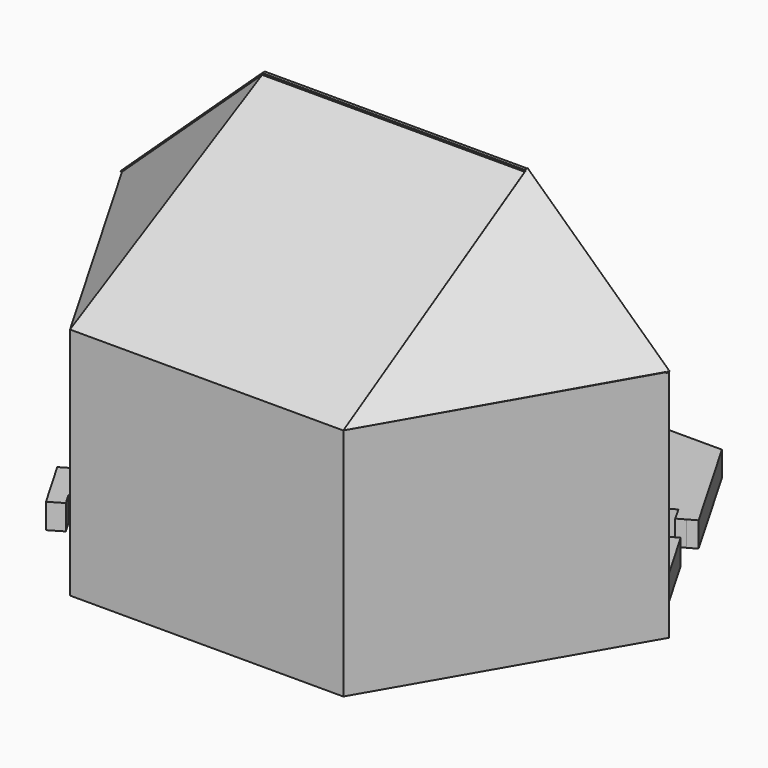
from build123d import *

# Parameters (mm, degrees)
F0_W      = 50
F0_H      = 12.5
F1_DEPTH  = 8
F2_DEPTH  = 75
F4_DEPTH  = 8
F7_DEPTH  = 3
F8_DEPTH  = 1
F11_DEPTH = 3
F14_DEPTH = 3
F15_DEPTH = 8
F16_DEPTH = 8


# Not quite as in the source:
# - a feature names something its author has since deleted; it is built from what else it names


with BuildPart() as f1:
    # F0 (on Top) → F1 (new body)
    with BuildSketch(Plane.XY):
        Polygon((57.9695070384, 39.3207329262), (60.5095952989, 40.7487522591), (42.0179491924, 72.7772228311), (-42.0179491924, 72.7772228311), (-84.0358983849, 0), (-42.0179491924, -72.7772228311), (42.0179491924, -72.7772228311), (84.0358983849, 0), (65.5097997054, 32.0881441788), (62.870004896, 30.6039762231), (65.3204122546, 26.2455930623), (60.0654171506, 23.2910848888), (57.615009792, 27.6494680496), (55.164720758, 32.0079177338), (52.7144317239, 36.366367418), (50.2642610162, 40.7248836223), (55.5194165334, 43.6791064608), align=None)
        with Locations((0, 54.5829171234)):
            Rectangle(F0_W, F0_H, mode=Mode.SUBTRACT)
    extrude(amount=F1_DEPTH)

    # F0 (on Top) → F2 (join)
    with BuildSketch(Plane.XY):
        Polygon((-84.0358983849, 0), (-87.5, 0), (-68.1246734519, -33.5590499945), (-63.1251610364, -42.2184595112), (-43.75, -75.7772228311), (43.75, -75.7772228311), (87.5, 0), (84.0358983849, 0), (42.0179491924, -72.7772228311), (-42.0179491924, -72.7772228311), align=None)
    extrude(amount=F2_DEPTH)

    # F0 (on Top) → F4 (join)
    with BuildSketch(Plane.XY):
        Polygon((43.75, 75.7772228311), (-43.75, 75.7772228311), (-65.625, 37.8886114156), (-68.125, 33.5584843966), (-87.5, 0), (-84.0358983849, 0), (-42.0179491924, 72.7772228311), (42.0179491924, 72.7772228311), (60.5095952989, 40.7487522591), (63.1248363216, 42.2190219338), align=None)
    extrude(amount=F4_DEPTH)

    # F6 (on face) → F7 (join)
    with BuildSketch(Plane(origin=(0, -50.1312366318, 89.3836679776), x_dir=(1, 0, 0), z_dir=(0, 0.4891706574, -0.872188092))):
        Polygon((43.75, 29.4041920927), (0, 29.4041920927), (-43.75, 29.4041920927), (-42.01795, -57.4775522498), (42.01795, -57.4775522498), align=None)
    extrude(amount=F7_DEPTH)

    # F3 (on Front) → F8 (join)
    with BuildSketch(Plane.XZ):
        Polygon((-42.01795, 114.5), (0, 114.5), (42.01795, 114.5), (84.0359, 75), (87.5, 75), (42.01795, 117.5), (0, 117.5), (-42.01795, 117.5), (-87.5, 75), (-84.0359, 75), align=None)
    extrude(amount=F8_DEPTH)

    # F10 (on face) → F11 (join)
    with BuildSketch(Plane(origin=(-67.6846727043, -39.0777640058, 72.4338274863), x_dir=(0.7723629594, -0.3015876344, 0.5590173143), z_dir=(-0.6351814378, -0.3667221741, 0.6797495039))):
        Polygon((33.2314262259, 55.789645187), (-25.6554603702, 35.6104118215), (30.9888924807, -31.0804218073), align=None)
    extrude(amount=-F11_DEPTH)

    # F13 (on face) → F14 (join)
    with BuildSketch(Plane(origin=(67.6756688636, -39.5950852503, 72.4241918832), x_dir=(0.7733047167, 0.3041472681, -0.556322078), z_dir=(-0.6340345536, 0.3709553614, -0.6785221475))):
        Polygon((-30.939509805, 30.5117392321), (-32.8751652468, -56.3649154418), (25.9400068576, -35.9776056011), align=None)
    extrude(amount=F14_DEPTH)

    # F0 (on Top) → F15 (join)
    with BuildSketch(Plane.XY):
        with Locations((0, 54.5829171234)):
            Rectangle(F0_W, F0_H)
    extrude(amount=F15_DEPTH)

    # F0 (on Top) → F16 (join)
    with BuildSketch(Plane.XY):
        Polygon((-77.8456264388, -39.3203929827), (-73.5443198074, -36.7711261738), (-75.8386599429, -32.8999502926), (-80.1399666105, -35.4492170403), align=None)
        Polygon((-63.1251610364, -42.2184595112), (-68.1246734519, -33.5590499945), (-73.5443198074, -36.7711261738), (-77.8456264388, -39.3203929827), (-72.8456167613, -47.9806414332), (-68.5445301574, -45.4310034146), align=None)
        Polygon((-66.2498559406, -49.3019813581), (-68.5445301574, -45.4310034146), (-72.8456167613, -47.9806414332), (-70.5509425445, -51.8516193767), align=None)
    extrude(amount=F16_DEPTH)


solid = f1.part
